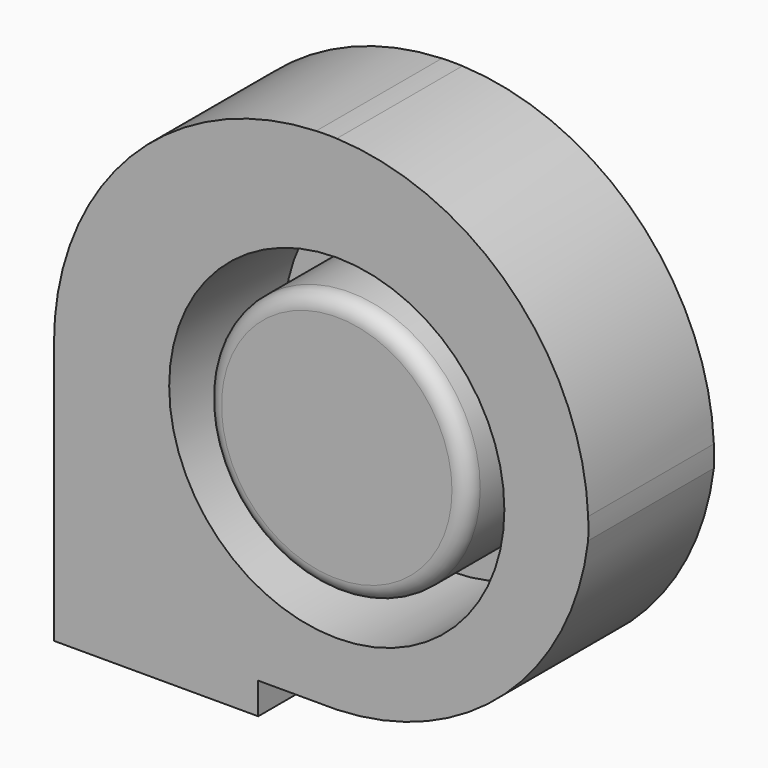
from build123d import *

# Parameters (mm, degrees)
F0_R     = 16
F1_DEPTH = 15
F0_R_2   = 12.5
F2_DEPTH = 1.25
F3_W     = 17
F3_H     = 12.5
F4_DEPTH = 10
F5_R     = 1.5


with BuildPart() as f1:
    # F0 (on Front) → F1 (new body)
    with BuildSketch(Plane.XZ):
        with BuildLine():
            Line((0, 25), (0, 0))
            Line((0, 0), (19.5, 0))
            Line((19.5, 0), (19.5, 3))
            Line((19.5, 3), (27, 3))
            ThreePointArc((27, 3), (43.0721423298, 9.5576629129), (51, 25))
            Line((51, 25), (51, 27.0383693291))
            ThreePointArc((51, 27.0383693291), (43.6843051192, 43.7109906775), (27, 51))
            Line((27, 51), (25.037037037, 51))
            ThreePointArc((25.037037037, 51), (7.2768537045, 43.0475290801), (0, 25))
        make_face()
        with Locations((27, 25)):
            Circle(F0_R, mode=Mode.SUBTRACT)
        with BuildLine():
            ThreePointArc((27, 51), (26.0185185185, 51.0185185185), (25.037037037, 51))
            Line((25.037037037, 51), (27, 51))
        make_face()
        with BuildLine():
            Line((51, 27.0383693291), (51, 25))
            ThreePointArc((51, 25), (51.0207833866, 26.0191846645), (51, 27.0383693291))
        make_face()
    extrude(amount=F1_DEPTH)



with BuildPart() as f1b:
    # F0 (on Front) → F1, piece 2 (new body)
    with BuildSketch(Plane.XZ):
        with Locations((27, 25)):
            Circle(F0_R_2)
    extrude(amount=F1_DEPTH)


with BuildPart() as f1_1:
    add(f1.part)

    add(f1b.part)  # F2 merges F1b
    # F0 (on Front) → F2 (join)
    with BuildSketch(Plane.XZ):
        with Locations((27, 25)):
            Circle(F0_R)
        with Locations((27, 25)):
            Circle(F0_R_2, mode=Mode.SUBTRACT)
    extrude(amount=F2_DEPTH)

    # F3 (on face) → F4 (cut)
    with BuildSketch(Plane(origin=(0, 0, 0), x_dir=(1, 0, 0), z_dir=(0, 0, -1))):
        with Locations((9.75, 7.5)):
            Rectangle(F3_W, F3_H)
    extrude(amount=-F4_DEPTH, mode=Mode.SUBTRACT)

    # F5
    f5_edges = [f1_1.edges().sort_by_distance(p)[0] for p in [
        (14.5, -15, 25),
    ]]
    fillet(f5_edges, radius=F5_R)


solid = f1_1.part
